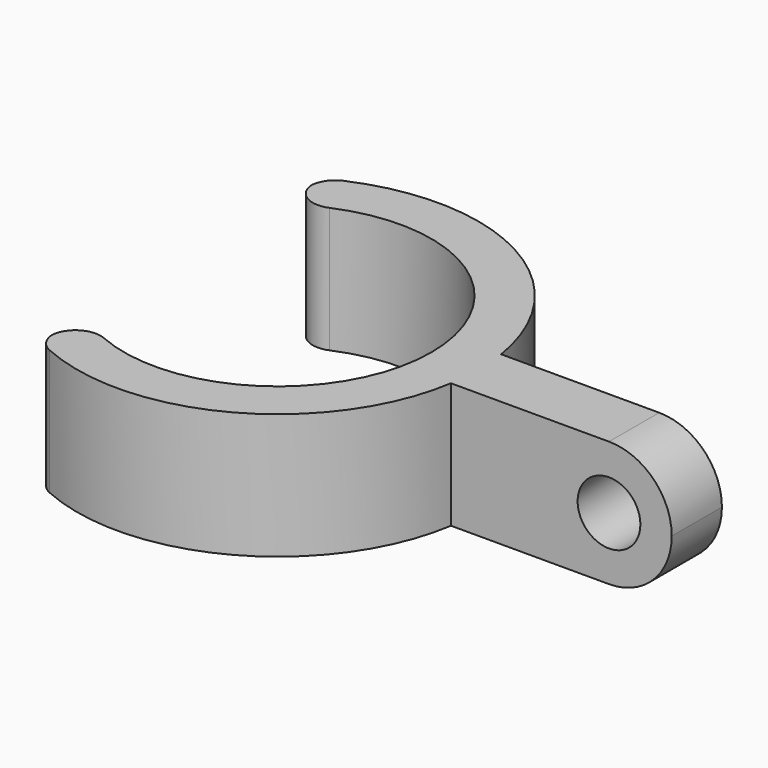
from build123d import *

# Parameters (mm, degrees)
F0_R        = 16
F0_R_2      = 12.25
F1_DEPTH    = 10
F2_W        = 11.453170795
F2_H        = 32.4866687879
F3_DEPTH    = 10.001
F4_T1_DEPTH = 27.6008886653
F4_T3_DEPTH = 16.6375565979
F5_W        = 20
F5_H        = 5
F6_DEPTH    = 10
F7_R        = 2.5
F8_DEPTH    = 18.501
F9_R        = 4.99999


# Not quite as in the source:
# - a fillet or chamfer that OpenCascade refuses, or shapes differently, is made with other operations: its cross-section is extruded or revolved along the edge and cut away or added
# - a fillet or chamfer is up to 0.001 mm smaller than in the source, because OpenCascade refuses the exact size


with BuildPart() as f1:
    # F0 (on Top) → F1 (new body)
    with BuildSketch(Plane.XY):
        Circle(F0_R)
        Circle(F0_R_2, mode=Mode.SUBTRACT)
    extrude(amount=F1_DEPTH)

    # F2 (on face) → F3 (cut, through all)
    with BuildSketch(Plane.XY.offset(10)):
        with Locations((-13.3922861423, 0.2399678342)):
            Rectangle(F2_W, F2_H)
    extrude(amount=-F3_DEPTH, mode=Mode.SUBTRACT)

    # F4: fillet of radius 2 on 4 edges, made by hand

    # F4_s2 → F4_t1 (cut)
    with BuildSketch(Plane.XY.offset(-8.8004443327)):
        with BuildLine():
            ThreePointArc((-7.6657007448, 13.0752565967), (-6.7633409093, 11.4033755993), (-4.8705146754, 11.2401328638))
            ThreePointArc((-4.8705146754, 11.2401328638), (-6.3244783193, 10.491114049), (-7.6657007448, 9.5550788637))
            Line((-7.6657007448, 9.5550788637), (-7.6657007448, 13.0752565967))
        make_face()
        with BuildLine():
            ThreePointArc((-4.8705146754, -11.2401328638), (-6.7633409093, -11.4033755993), (-7.6657007448, -13.0752565967))
            Line((-7.6657007448, -13.0752565967), (-7.6657007448, -9.5550788637))
            ThreePointArc((-7.6657007448, -9.5550788637), (-6.3244783193, -10.491114049), (-4.8705146754, -11.2401328638))
        make_face()
    extrude(amount=F4_T1_DEPTH, mode=Mode.SUBTRACT)

    # F4_s4 → F4_t3 (cut)
    with BuildSketch(Plane.XY.offset(-3.318778299)):
        with BuildLine():
            ThreePointArc((-6.4750865655, -14.6312423932), (-7.3418230019, -13.8934897778), (-7.6657007448, -12.8023370941))
            Line((-7.6657007448, -12.8023370941), (-7.6657007448, -14.0441102278))
            ThreePointArc((-7.6657007448, -14.0441102278), (-7.076485532, -14.3500297044), (-6.4750865655, -14.6312423932))
        make_face()
        with BuildLine():
            ThreePointArc((-6.4750865655, 14.6312423932), (-7.3418230019, 13.8934897778), (-7.6657007448, 12.8023370941))
            Line((-7.6657007448, 12.8023370941), (-7.6657007448, 14.0441102278))
            ThreePointArc((-7.6657007448, 14.0441102278), (-7.076485532, 14.3500297044), (-6.4750865655, 14.6312423932))
        make_face()
    extrude(amount=F4_T3_DEPTH, mode=Mode.SUBTRACT)

    # F5 (on face) → F6 (join)
    with BuildSketch(Plane.XY.offset(10)):
        with Locations((23.4022848308, 0)):
            Rectangle(F5_W, F5_H)
    extrude(amount=-F6_DEPTH)

    # F7 (on face) → F8 (cut, through all)
    with BuildSketch(Plane.XZ.offset(2.5)):
        with Locations((28.4022848308, 5)):
            Circle(F7_R)
    extrude(amount=-F8_DEPTH, mode=Mode.SUBTRACT)

    # F9 (radius 5 in the source; OpenCascade refuses exactly that, so slightly less here)
    f9_edges = [f1.edges().sort_by_distance(p)[0] for p in [
        (33.402285, 0, 10),
        (33.402285, 0, 0),
    ]]
    fillet(f9_edges, radius=F9_R)


solid = f1.part
